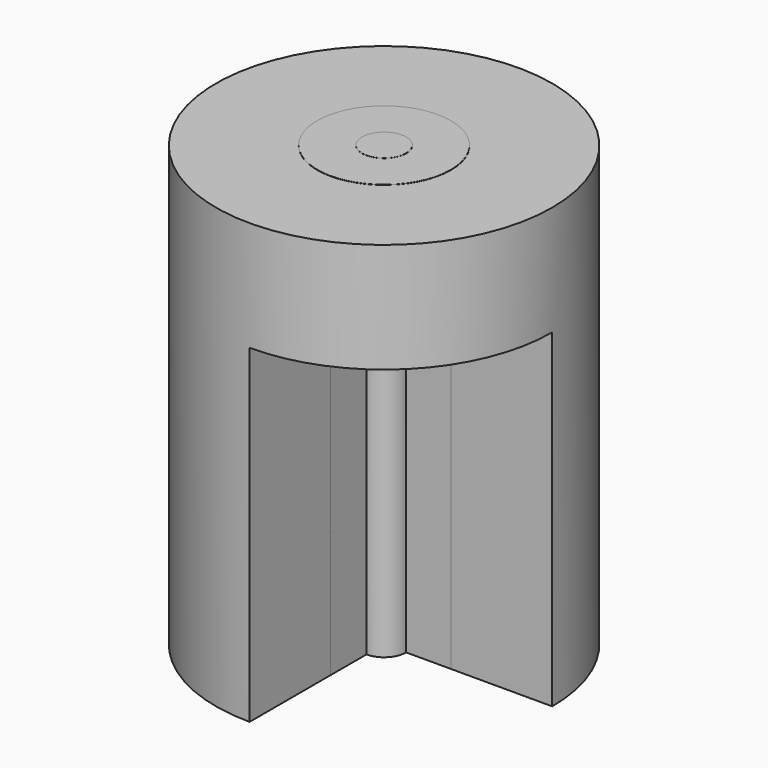
from build123d import *

# Parameters (mm, degrees)
F0_R     = 194.5330357486
F3_DEPTH = 508
F1_R     = 77.2129975411
F4_DEPTH = 508.254
F2_R     = 25.5304809281
F5_DEPTH = 508.381
F7_DEPTH = 381


with BuildPart() as f3:
    # F0 (on Top) → F3 (new body)
    with BuildSketch(Plane.XY):
        Circle(F0_R)
    extrude(amount=F3_DEPTH)


with BuildPart() as f4:
    # F1 (on Top) → F4 (new body)
    with BuildSketch(Plane.XY):
        Circle(F1_R)
    extrude(amount=F4_DEPTH)


with BuildPart() as f5:
    # F2 (on Top) → F5 (new body)
    with BuildSketch(Plane.XY):
        Circle(F2_R)
    extrude(amount=F5_DEPTH)


with BuildPart() as f7_tool:
    # F6 (on Top) → F7 (new body)
    with BuildSketch(Plane.XY):
        with BuildLine():
            Line((257.4372589588, 0), (0, 0))
            Line((0, 0), (0, -257.4372589588))
            ThreePointArc((0, -257.4372589588), (182.0356315399, -182.0356315399), (257.4372589588, 0))
        make_face()
    extrude(amount=F7_DEPTH)


with BuildPart() as f3_1:
    add(f3.part)

    # F7: cut by f7_tool
    add(f7_tool.part, mode=Mode.SUBTRACT)


with BuildPart() as f4_1:
    add(f4.part)

    # F7: cut by f7_tool
    add(f7_tool.part, mode=Mode.SUBTRACT)


solid = Compound([f5.part, f3_1.part, f4_1.part])
